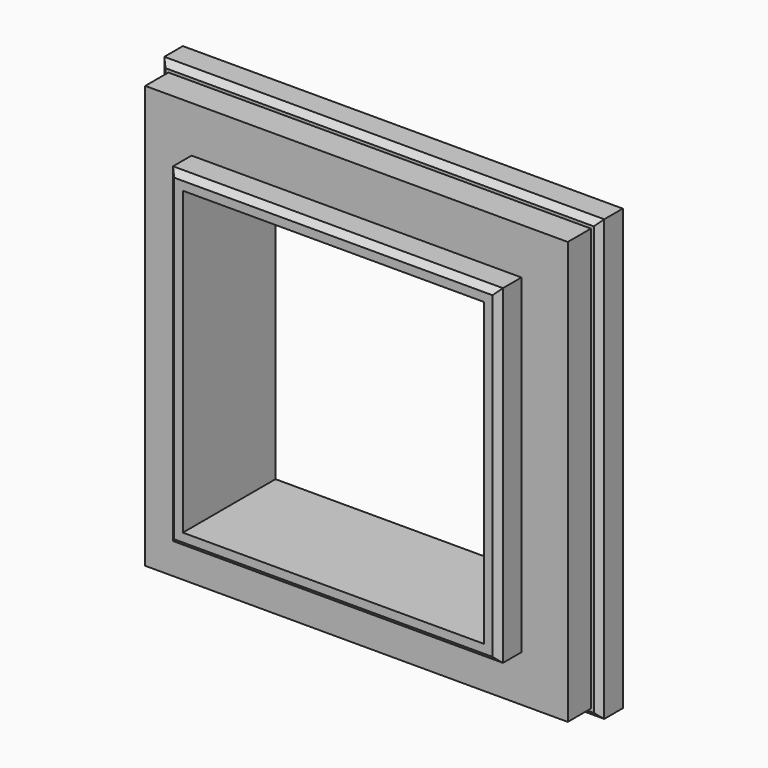
from build123d import *

# Parameters (mm, degrees)
F0_W          = 73
F0_H          = 73
F0_W_2        = 56
F0_H_2        = 56
F0_W_3        = 52
F0_H_3        = 52
F1_DEPTH      = 20
F0_W_4        = 76
F0_H_4        = 76
F2_DEPTH      = 3
F3_DEPTH      = 10
F4_W          = 10
F4_H          = 5
F5_DEPTH      = 80
F6_W          = 5
F6_H          = 10
F7_DEPTH      = 80
F8_W          = 8
F8_H          = 5
F9_DEPTH      = 80
F10_W         = 5
F10_H         = 8
F11_DEPTH     = 80
F12_SIZE      = 1
F13_T         = 2.5
F13_T3_DEPTH  = 62
F13_T5_DEPTH  = 62
F13_T7_DEPTH  = 78
F13_T9_DEPTH  = 78
F13_T11_DEPTH = 25


# Not quite as in the source:
# - a shell that OpenCascade refuses in one call is made with other operations: the cavity is built on its own and cut out


with BuildPart() as f1:
    # F0 (on Front) → F1 (new body)
    with BuildSketch(Plane.XZ):
        with Locations((38, 38)):
            Rectangle(F0_W, F0_H)
        with Locations((38, 38)):
            Rectangle(F0_W_2, F0_H_2, mode=Mode.SUBTRACT)
        with Locations((38, 38)):
            Rectangle(F0_W_2, F0_H_2)
        with Locations((38, 38)):
            Rectangle(F0_W_3, F0_H_3, mode=Mode.SUBTRACT)
    extrude(amount=F1_DEPTH)

    # F0 (on Front) → F2 (join)
    with BuildSketch(Plane.XZ):
        with Locations((38, 38)):
            Rectangle(F0_W_4, F0_H_4)
        with Locations((38, 38)):
            Rectangle(F0_W, F0_H, mode=Mode.SUBTRACT)
    extrude(amount=F2_DEPTH)

    # F0 (on Front) → F3 (join)
    with BuildSketch(Plane.XZ):
        with Locations((38, 38)):
            Rectangle(F0_W_4, F0_H_4)
        with Locations((38, 38)):
            Rectangle(F0_W, F0_H, mode=Mode.SUBTRACT)
    extrude(amount=F3_DEPTH)

    # F4 (on Top) → F5 (cut)
    with BuildSketch(Plane.XY):
        with Locations((5, -2.5)):
            Rectangle(F4_W, F4_H)
        with Locations((71, -2.5)):
            Rectangle(F4_W, F4_H)
    extrude(amount=F5_DEPTH, mode=Mode.SUBTRACT)

    # F6 (on Right) → F7 (cut)
    with BuildSketch(Plane.YZ):
        with Locations((-2.5, 5)):
            Rectangle(F6_W, F6_H)
        with Locations((-2.5, 71)):
            Rectangle(F6_W, F6_H)
    extrude(amount=F7_DEPTH, mode=Mode.SUBTRACT)

    # F8 (on Top) → F9 (cut)
    with BuildSketch(Plane.XY):
        with Locations((5.5, -17.5)):
            Rectangle(F8_W, F8_H)
        with Locations((70.5, -17.5)):
            Rectangle(F8_W, F8_H)
    extrude(amount=F9_DEPTH, mode=Mode.SUBTRACT)

    # F10 (on Right) → F11 (cut)
    with BuildSketch(Plane.YZ):
        with Locations((-17.5, 5.5)):
            Rectangle(F10_W, F10_H)
        with Locations((-17.5, 70.5)):
            Rectangle(F10_W, F10_H)
    extrude(amount=F11_DEPTH, mode=Mode.SUBTRACT)

    # F12
    f12_edges = [f1.edges().sort_by_distance(p)[0] for p in [
        (38, -10, 0),
        (0, -10, 38),
        (76, -10, 38),
        (38, -10, 76),
        (66.5, -20, 38),
        (38, -20, 66.5),
        (38, -20, 9.5),
        (9.5, -20, 38),
    ]]
    chamfer(f12_edges, length=F12_SIZE)

    # F13: shell of thickness 2.5, made by hand


with BuildPart() as f13_core1:
    # F13_t2: copy of F1
    add(f1.part)

    # the walls: a layer under each face that stays
    f13_faces = [f13_core1.faces().sort_by_distance(p)[0] for p in [
        (9.5, -17, 38),
        (38, -17, 66.5),
        (10, -19.5, 38),
        (69.2857142857, -15, 69.2857142857),
        (38, -17, 9.5),
        (38, -19.5, 66),
        (66.5, -17, 38),
        (38, -19.5, 10),
        (56.90625, -20, 11.1790123457),
        (1.5, -12.5, 38),
        (38, -12.5, 1.5),
        (74.5, -12.5, 38),
        (38, -12.5, 74.5),
        (66, -19.5, 38),
        (64, -10, 38),
        (38, -10, 64),
        (38, -10, 12),
        (12, -10, 38),
        (40.890625, -10, 1.304526749),
        (11.8666666667, 0, 11.8666666667),
        (38, -9.5, 0.5),
        (0.5, -9.5, 38),
        (75.5, -9.5, 38),
        (38, -9.5, 75.5),
        (66, -2.5, 38),
        (38, -2.5, 10),
        (10, -2.5, 38),
        (38, -2.5, 66),
        (38, -7, 0),
        (0, -7, 38),
        (76, -7, 38),
        (38, -7, 76),
    ]]
    thicken(f13_faces, amount=-F13_T, mode=Mode.SUBTRACT)

    # F13_s4 → F13_t3 (cut)
    with BuildSketch(Plane.XY.offset(7)):
        Polygon((9.475, -15.025), (12, -15), (12, -12.5), (9.5, -12.5), align=None)
        Polygon((66.525, -15.025), (66.5, -12.5), (64, -12.5), (64, -15), align=None)
    extrude(amount=F13_T3_DEPTH, mode=Mode.SUBTRACT)

    # F13_s6 → F13_t5 (cut)
    with BuildSketch(Plane.YZ.offset(7)):
        Polygon((-15.025, 66.525), (-15, 64), (-12.5, 64), (-12.5, 66.5), align=None)
        Polygon((-15.025, 9.475), (-12.5, 9.5), (-12.5, 12), (-15, 12), align=None)
    extrude(amount=F13_T5_DEPTH, mode=Mode.SUBTRACT)

    # F13_s8 → F13_t7 (cut)
    with BuildSketch(Plane.XY.offset(-1)):
        Polygon((1.475, -10.025), (4, -10), (4, -7.5), (1.5, -7.5), align=None)
        Polygon((74.525, -10.025), (72, -10), (72, -7.5), (74.5, -7.5), align=None)
    extrude(amount=F13_T7_DEPTH, mode=Mode.SUBTRACT)

    # F13_s10 → F13_t9 (cut)
    with BuildSketch(Plane.YZ.offset(-1)):
        Polygon((-10.025, 1.475), (-10, 4), (-7.5, 4), (-7.5, 1.5), align=None)
        Polygon((-10.025, 74.525), (-10, 72), (-7.5, 72), (-7.5, 74.5), align=None)
    extrude(amount=F13_T9_DEPTH, mode=Mode.SUBTRACT)

    # F13_s12 → F13_t11 (cut)
    with BuildSketch(Plane.XZ.offset(-2.5)):
        Polygon((63.975, 63.975), (66.5, 64), (66.5, 66.5), (64, 66.5), align=None)
        Polygon((63.975, 12.025), (66.5, 12), (66.5, 9.5), (64, 9.5), align=None)
        Polygon((12.025, 63.975), (12, 66.5), (9.5, 66.5), (9.5, 64), align=None)
        Polygon((12.025, 12.025), (12, 9.5), (9.5, 9.5), (9.5, 12), align=None)
    extrude(amount=F13_T11_DEPTH, mode=Mode.SUBTRACT)


with BuildPart() as f1_1:
    add(f1.part)

    # what is left inside the walls is the cavity
    f13_cavity = [f13_core1.part.solids().sort_by_distance(p)[0] for p in [
        (65.611111, -5.025, 6.9375),
    ]]
    add(f13_cavity, mode=Mode.SUBTRACT)


solid = f1_1.part
